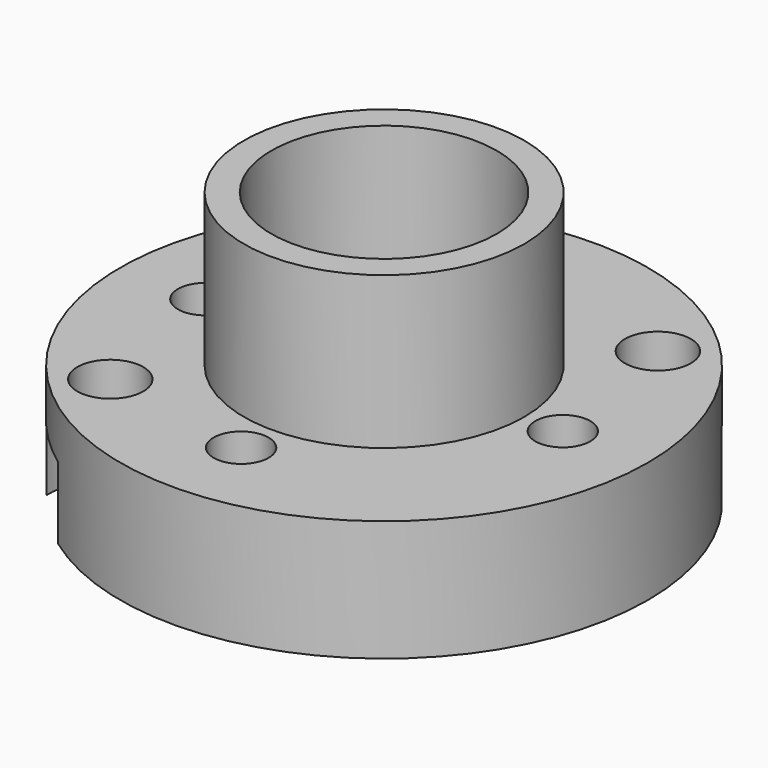
from build123d import *

# Parameters (mm, degrees)
F0_R     = 6.375
F0_R_2   = 5.125
F1_DEPTH = 6.92
F0_R_3   = 12
F0_R_4   = 1.5
F0_R_5   = 1.25
F2_DEPTH = 5.5
F5_DEPTH = 3.27
F6_DEPTH = 5.5


with BuildPart() as f1:
    # F0 (on Top) → F1 (new body)
    with BuildSketch(Plane.XY):
        Circle(F0_R)
        Circle(F0_R_2, mode=Mode.SUBTRACT)
    extrude(amount=F1_DEPTH)


with BuildPart() as f2:
    # F0 (on Top) → F2 (new body)
    with BuildSketch(Plane.XY):
        Circle(F0_R_3)
        with Locations((-6.91550432, -6.91550432)):
            Circle(F0_R_4, mode=Mode.SUBTRACT)
        with Locations((0, -8.125)):
            Circle(F0_R_5, mode=Mode.SUBTRACT)
        with Locations((-8.125, 0)):
            Circle(F0_R_5, mode=Mode.SUBTRACT)
        Circle(F0_R, mode=Mode.SUBTRACT)
        with Locations((8.125, 0)):
            Circle(F0_R_5, mode=Mode.SUBTRACT)
        with Locations((0, 8.125)):
            Circle(F0_R_5, mode=Mode.SUBTRACT)
        with Locations((6.91550432, 6.91550432)):
            Circle(F0_R_4, mode=Mode.SUBTRACT)
    extrude(amount=-F2_DEPTH)

    # F4 (on offset) → F5 (cut)
    with BuildSketch(Plane(origin=(0, 0, -5.5), x_dir=(1, 0, 0), z_dir=(0, 0, -1))):
        with BuildLine():
            ThreePointArc((-9.7123834889, 7.0476667745), (-4.9356053327, 4.9356053327), (-7.0476667745, 9.7123834889))
            ThreePointArc((-7.0476667745, 9.7123834889), (-8.4852813742, 8.4852813742), (-9.7123834889, 7.0476667745))
        make_face()
        with BuildLine():
            ThreePointArc((7.0476667745, -9.7123834889), (8.4852813742, -8.4852813742), (9.7123834889, -7.0476667745))
            ThreePointArc((9.7123834889, -7.0476667745), (4.9356053327, -4.9356053327), (7.0476667745, -9.7123834889))
        make_face()
    extrude(amount=-F5_DEPTH, mode=Mode.SUBTRACT)


with BuildPart() as f6:
    # F0 (on Top) → F6 (new body)
    with BuildSketch(Plane.XY):
        Circle(F0_R)
        Circle(F0_R_2, mode=Mode.SUBTRACT)
    extrude(amount=-F6_DEPTH)


solid = Compound([f1.part, f2.part, f6.part])
